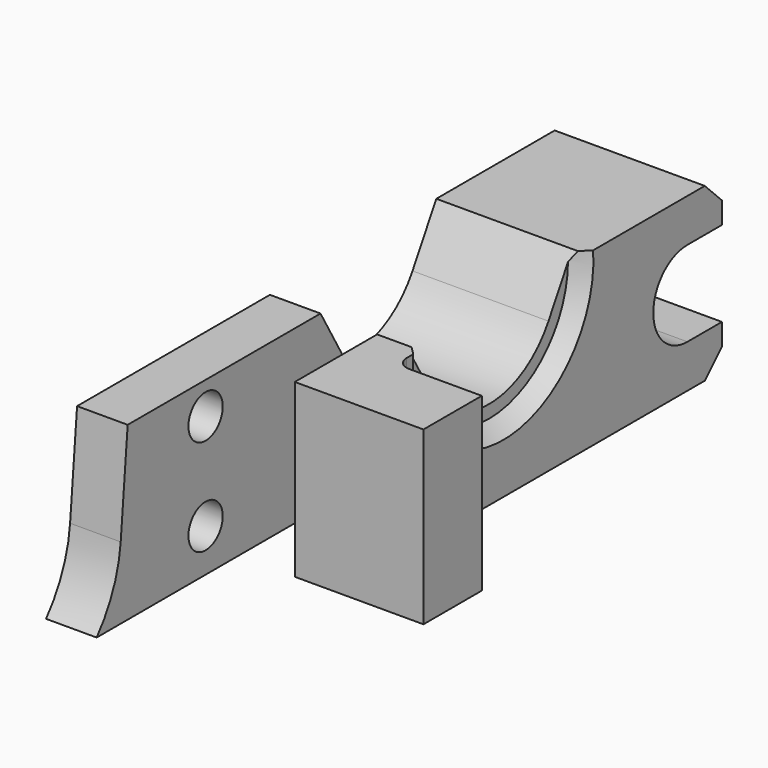
from build123d import *

# Parameters (mm, degrees)
F1_DEPTH  = 50.8
F2_R      = 3.9624
F3_SIZE   = 6.35
F5_DEPTH  = 44.451
F7_D      = 13.0302
F9_DEPTH  = 69.851
F10_R     = 29.21
F11_DEPTH = 29.591
F12_SIZE  = 4.19099
F14_DEPTH = 14.9870001
F16_DEPTH = 16.764
F17_R     = 6.35
F18_DEPTH = 69.851


# Not quite as in the source:
# - a fillet or chamfer is up to 0.001 mm smaller than in the source, because OpenCascade refuses the exact size


with BuildPart() as f1:
    # F0 (on Top) → F1 (new body)
    with BuildSketch(Plane.XY):
        Polygon((44.45, 120.65), (0, 120.65), (0, 0), (0, -21.59), (0, -73.9648), (14.986, -73.9648), (14.986, 26.2809675187), (31.75, 26.2809675187), (31.75, -21.59), (69.85, -21.59), (69.85, 0), (44.45, 0), align=None)
    extrude(amount=F1_DEPTH)

    # F2
    f2_edges = [f1.edges().sort_by_distance(p)[0] for p in [
        (44.45, 0, 25.4),
        (14.986, 26.280968, 25.4),
        (31.75, 26.280968, 25.4),
    ]]
    fillet(f2_edges, radius=F2_R)

    # F3
    f3_edges = [f1.edges().sort_by_distance(p)[0] for p in [
        (22.225, 120.65, 50.8),
        (22.225, 120.65, 0),
    ]]
    chamfer(f3_edges, length=F3_SIZE)

    # F4 (on face) → F5 (cut, through all)
    with BuildSketch(Plane.YZ.offset(44.45)):
        with BuildLine():
            Line((120.65, 38.0365), (107.8865, 38.0365))
            ThreePointArc((107.8865, 38.0365), (95.25, 25.4), (107.8865, 12.7635))
            Line((107.8865, 12.7635), (120.65, 12.7635))
            Line((120.65, 12.7635), (120.65, 38.0365))
        make_face()
    extrude(amount=-F5_DEPTH, mode=Mode.SUBTRACT)

    # F7 (through all)
    with Locations(Plane.YZ.offset(69.85)):
        with Locations((7.62, 12.954)):
            Hole(F7_D / 2)

    # F8 (on face) → F9 (cut, through all)
    with BuildSketch(Plane(origin=(0, 0, 0), x_dir=(0, -1, 0), z_dir=(-1, 0, 0))):
        with BuildLine():
            Line((-8.8916366414, 50.8), (-70.4833633586, 50.8))
            Line((-70.4833633586, 50.8), (-61.6845452561, 35.56))
            ThreePointArc((-61.6845452561, 35.56), (-39.6875, 22.86), (-17.6904547439, 35.56))
            Line((-17.6904547439, 35.56), (-8.8916366414, 50.8))
        make_face()
    extrude(amount=-F9_DEPTH, mode=Mode.SUBTRACT)

    # F10 (on face) → F11 (cut)
    with BuildSketch(Plane.YZ.offset(69.85)):
        with Locations((39.6875, 48.26)):
            Circle(F10_R)
    extrude(amount=-F11_DEPTH, mode=Mode.SUBTRACT)

    # F12 (size 4.191 in the source; OpenCascade refuses exactly that, so slightly less here)
    f12_edges = [f1.edges().sort_by_distance(p)[0] for p in [
        (44.45, 39.6875, 19.05),
    ]]
    chamfer(f12_edges, length=F12_SIZE)

    # F13 (on face) → F14 (cut, through all)
    with BuildSketch(Plane.YZ.offset(14.986)):
        with BuildLine():
            Line((-73.9648, 50.8), (-73.9648, 0))
            ThreePointArc((-73.9648, 0), (-67.8661098873, 9.9669221787), (-65.0748, 21.3133818873))
            Line((-65.0748, 21.3133818873), (-62.4950551894, 50.8))
            Line((-62.4950551894, 50.8), (-73.9648, 50.8))
        make_face()
    extrude(amount=-F14_DEPTH, mode=Mode.SUBTRACT)

    # F15 (on face) → F16 (cut, through all)
    with BuildSketch(Plane.YZ.offset(14.986)):
        Polygon((11.9264439221, 19.6698105436), (22.8565887415, 19.6698105436), (41.9241071546, 38.7373289567), (11.9264439221, 38.7373289567), align=None)
    extrude(amount=F16_DEPTH, mode=Mode.SUBTRACT)

    # F17 (on face) → F18 (cut, through all)
    with BuildSketch(Plane(origin=(0, 0, 0), x_dir=(0, -1, 0), z_dir=(-1, 0, 0))):
        with Locations((33.655, 12.7)):
            Circle(F17_R)
        with Locations((33.655, 41.275)):
            Circle(F17_R)
    extrude(amount=-F18_DEPTH, mode=Mode.SUBTRACT)


solid = f1.part
